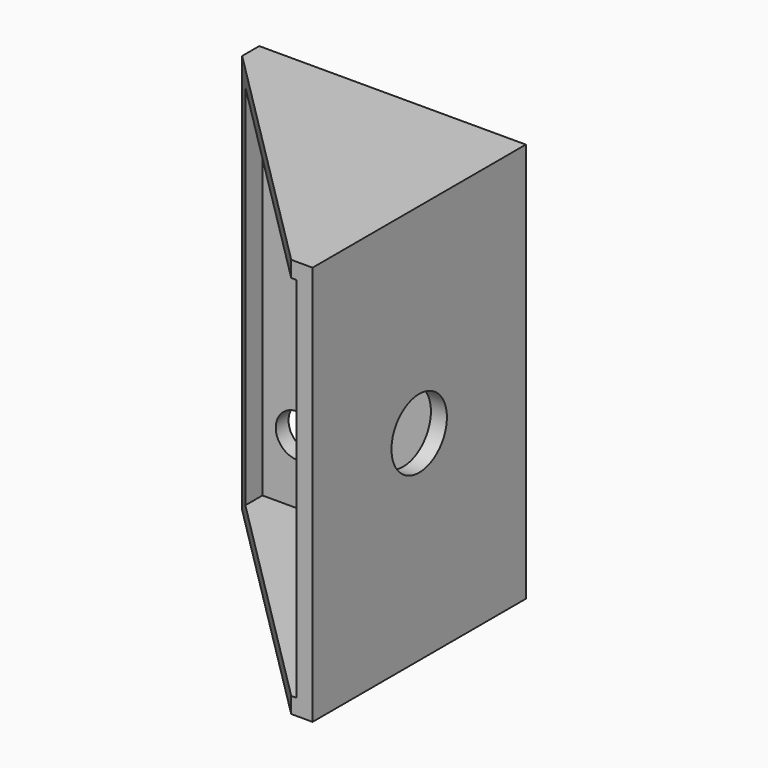
from build123d import *

# Parameters (mm, degrees)
F0_W        = 50
F0_H        = 75
F1_DEPTH    = 50
F2_W        = 44
F2_H        = 69
F3_DEPTH    = 47
F4_T1_DEPTH = 311.5948348929
F5_R        = 4
F5_R_2      = 2
F6_DEPTH    = 3
F7_R        = 6.5
F8_DEPTH    = 3


# Not quite as in the source:
# - a fillet or chamfer that OpenCascade refuses, or shapes differently, is made with other operations: its cross-section is extruded or revolved along the edge and cut away or added


with BuildPart() as f1:
    # F0 (on Front) → F1 (new body)
    with BuildSketch(Plane.XZ):
        Rectangle(F0_W, F0_H)
    extrude(amount=F1_DEPTH)

    # F2 (on face) → F3 (cut)
    with BuildSketch(Plane.XZ.offset(50)):
        Rectangle(F2_W, F2_H)
    extrude(amount=-F3_DEPTH, mode=Mode.SUBTRACT)

    # F4: chamfer of 46 on 1 edges, made by hand

    # F4_s2 → F4_t1 (cut)
    with BuildSketch(Plane.XY.offset(-155.7974174464)):
        Polygon((-25, -4), (21, -50), (-25, -50), align=None)
    extrude(amount=F4_T1_DEPTH, mode=Mode.SUBTRACT)

    # F5 (on face) → F6 (cut, through all)
    with BuildSketch(Plane.XZ.offset(3)):
        with Locations((-15.5, 22.5)):
            Circle(F5_R)
        with Locations((15.5, 22.5)):
            Circle(F5_R)
        with Locations((15.5, -22.5)):
            Circle(F5_R)
        with Locations((-15.5, -22.5)):
            Circle(F5_R)
        Circle(F5_R_2)
    extrude(amount=-F6_DEPTH, mode=Mode.SUBTRACT)

    # F7 (on face) → F8 (cut, through all)
    with BuildSketch(Plane.YZ.offset(25)):
        with Locations((-25, 0)):
            Circle(F7_R)
    extrude(amount=-F8_DEPTH, mode=Mode.SUBTRACT)


solid = f1.part
